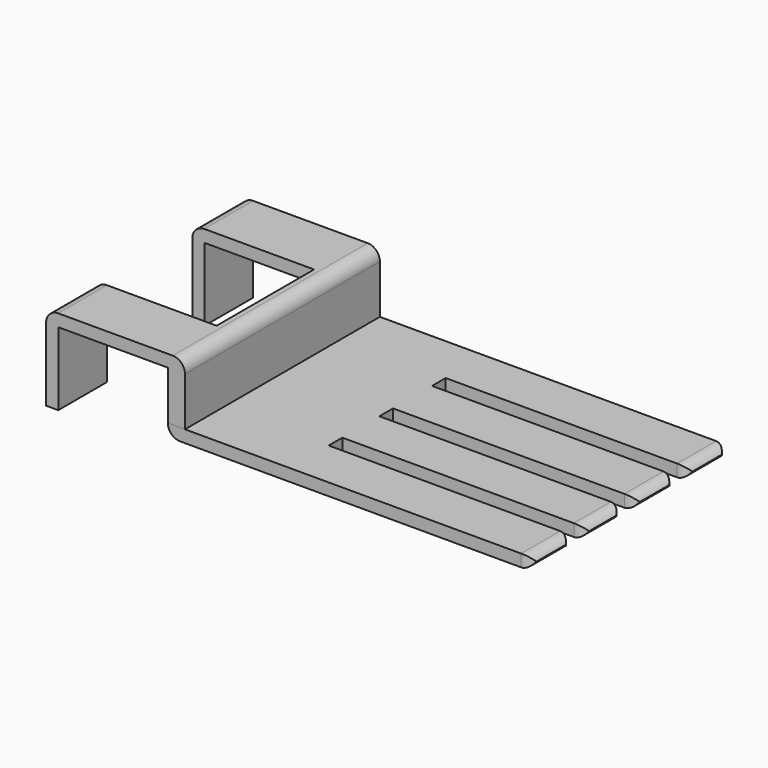
from build123d import *

# Parameters (mm, degrees)
F0_W         = 150
F0_H         = 100
F1_DEPTH     = 5
F2_W         = 100
F2_H         = 7
F3_DEPTH     = 5.001
F4_W         = 7
F4_H         = 100
F5_DEPTH     = 25
F6_W         = 25
F6_H         = 5
F7_DEPTH     = 50
F9_W         = 5
F9_H         = 25
F8_W         = 5
F8_H         = 25
F10_DEPTH    = 30
F11_R        = 4.99999
F11_2_R      = 4.99999
F12_T1_DEPTH = 45
F12_T3_DEPTH = 30
F12_T5_DEPTH = 44
F12_T7_DEPTH = 45
F12_T9_DEPTH = 45


# Not quite as in the source:
# - a fillet or chamfer that OpenCascade refuses, or shapes differently, is made with other operations: its cross-section is extruded or revolved along the edge and cut away or added
# - a fillet or chamfer is up to 0.001 mm smaller than in the source, because OpenCascade refuses the exact size


with BuildPart() as f1:
    # F0 (on Top) → F1 (new body)
    with BuildSketch(Plane.XY):
        with Locations((-2.425318882, 2.1896716207)):
            Rectangle(F0_W, F0_H)
    extrude(amount=F1_DEPTH)

    # F2 (on face) → F3 (cut, through all)
    with BuildSketch(Plane.XY.offset(5)):
        with Locations((22.574681118, 28.6896716207)):
            Rectangle(F2_W, F2_H)
        with Locations((22.574681118, 1.6896716207)):
            Rectangle(F2_W, F2_H)
        with Locations((22.574681118, -24.3103283793)):
            Rectangle(F2_W, F2_H)
    extrude(amount=-F3_DEPTH, mode=Mode.SUBTRACT)

    # F11#2 (radius 5 in the source; OpenCascade refuses exactly that, so slightly less here)
    f11_2_edges = [f1.edges().sort_by_distance(p)[0] for p in [
        (-77.425319, 2.189672, 0),
    ]]
    fillet(f11_2_edges, radius=F11_2_R)

    # F12: fillet of radius 5 on 16 edges, made by hand

    # F12_s2 → F12_t1 (cut)
    with BuildSketch(Plane.XZ.offset(15.3103283793)):
        with BuildLine():
            ThreePointArc((67.574681118, 0), (71.110215024, 1.4644660941), (72.574681118, 5))
            Line((72.574681118, 5), (72.574681118, 0))
            Line((72.574681118, 0), (67.574681118, 0))
        make_face()
        with BuildLine():
            ThreePointArc((67.574681118, 5), (71.110215024, 3.5355339059), (72.574681118, 0))
            Line((72.574681118, 0), (72.574681118, 5))
            Line((72.574681118, 5), (67.574681118, 5))
        make_face()
    extrude(amount=F12_T1_DEPTH, mode=Mode.SUBTRACT)

    # F12_s4 → F12_t3 (cut)
    with BuildSketch(Plane.XY.offset(-12.5)):
        with BuildLine():
            ThreePointArc((67.574681118, -27.8103283793), (71.110215024, -29.2747944733), (72.574681118, -32.8103283793))
            Line((72.574681118, -32.8103283793), (72.574681118, -27.8103283793))
            Line((72.574681118, -27.8103283793), (67.574681118, -27.8103283793))
        make_face()
        with BuildLine():
            ThreePointArc((67.574681118, -47.8103283793), (71.110215024, -46.3458622852), (72.574681118, -42.8103283793))
            Line((72.574681118, -42.8103283793), (72.574681118, -47.8103283793))
            Line((72.574681118, -47.8103283793), (67.574681118, -47.8103283793))
        make_face()
        with BuildLine():
            ThreePointArc((67.574681118, -1.8103283793), (71.110215024, -3.2747944733), (72.574681118, -6.8103283793))
            Line((72.574681118, -6.8103283793), (72.574681118, -1.8103283793))
            Line((72.574681118, -1.8103283793), (67.574681118, -1.8103283793))
        make_face()
        with BuildLine():
            ThreePointArc((72.574681118, -15.8103283793), (71.110215024, -19.3458622852), (67.574681118, -20.8103283793))
            Line((67.574681118, -20.8103283793), (72.574681118, -20.8103283793))
            Line((72.574681118, -20.8103283793), (72.574681118, -15.8103283793))
        make_face()
        with BuildLine():
            ThreePointArc((67.574681118, 25.1896716207), (71.110215024, 23.7252055267), (72.574681118, 20.1896716207))
            Line((72.574681118, 20.1896716207), (72.574681118, 25.1896716207))
            Line((72.574681118, 25.1896716207), (67.574681118, 25.1896716207))
        make_face()
        with BuildLine():
            ThreePointArc((72.574681118, 10.1896716207), (71.110215024, 6.6541377148), (67.574681118, 5.1896716207))
            Line((67.574681118, 5.1896716207), (72.574681118, 5.1896716207))
            Line((72.574681118, 5.1896716207), (72.574681118, 10.1896716207))
        make_face()
        with BuildLine():
            ThreePointArc((67.574681118, 52.1896716207), (71.110215024, 50.7252055267), (72.574681118, 47.1896716207))
            Line((72.574681118, 47.1896716207), (72.574681118, 52.1896716207))
            Line((72.574681118, 52.1896716207), (67.574681118, 52.1896716207))
        make_face()
        with BuildLine():
            ThreePointArc((72.574681118, 37.1896716207), (71.110215024, 33.6541377148), (67.574681118, 32.1896716207))
            Line((67.574681118, 32.1896716207), (72.574681118, 32.1896716207))
            Line((72.574681118, 32.1896716207), (72.574681118, 37.1896716207))
        make_face()
    extrude(amount=F12_T3_DEPTH, mode=Mode.SUBTRACT)

    # F12_s6 → F12_t5 (cut)
    with BuildSketch(Plane.XZ.offset(-10.6896716207)):
        with BuildLine():
            ThreePointArc((67.574681118, 0), (71.110215024, 1.4644660941), (72.574681118, 5))
            Line((72.574681118, 5), (72.574681118, 0))
            Line((72.574681118, 0), (67.574681118, 0))
        make_face()
        with BuildLine():
            ThreePointArc((67.574681118, 5), (71.110215024, 3.5355339059), (72.574681118, 0))
            Line((72.574681118, 0), (72.574681118, 5))
            Line((72.574681118, 5), (67.574681118, 5))
        make_face()
    extrude(amount=F12_T5_DEPTH, mode=Mode.SUBTRACT)

    # F12_s8 → F12_t7 (cut)
    with BuildSketch(Plane.XZ.offset(-37.6896716207)):
        with BuildLine():
            ThreePointArc((67.574681118, 0), (71.110215024, 1.4644660941), (72.574681118, 5))
            Line((72.574681118, 5), (72.574681118, 0))
            Line((72.574681118, 0), (67.574681118, 0))
        make_face()
        with BuildLine():
            ThreePointArc((67.574681118, 5), (71.110215024, 3.5355339059), (72.574681118, 0))
            Line((72.574681118, 0), (72.574681118, 5))
            Line((72.574681118, 5), (67.574681118, 5))
        make_face()
    extrude(amount=F12_T7_DEPTH, mode=Mode.SUBTRACT)

    # F12_s10 → F12_t9 (cut)
    with BuildSketch(Plane.XZ.offset(-64.6896716207)):
        with BuildLine():
            ThreePointArc((67.574681118, 0), (71.110215024, 1.4644660941), (72.574681118, 5))
            Line((72.574681118, 5), (72.574681118, 0))
            Line((72.574681118, 0), (67.574681118, 0))
        make_face()
        with BuildLine():
            ThreePointArc((67.574681118, 5), (71.110215024, 3.5355339059), (72.574681118, 0))
            Line((72.574681118, 0), (72.574681118, 5))
            Line((72.574681118, 5), (67.574681118, 5))
        make_face()
    extrude(amount=F12_T9_DEPTH, mode=Mode.SUBTRACT)


with BuildPart() as f5:
    # F4 (on face) → F5 (new body)
    with BuildSketch(Plane.XY.offset(5)):
        with Locations((-73.925318882, 2.1896716207)):
            Rectangle(F4_W, F4_H)
    extrude(amount=F5_DEPTH)

    # F6 (on face) → F7 (join)
    with BuildSketch(Plane(origin=(-77.425318882, 0, 0), x_dir=(0, -1, 0), z_dir=(-1, 0, 0))):
        with Locations((-39.6896716207, 27.5)):
            Rectangle(F6_W, F6_H)
        with Locations((35.3103283793, 27.5)):
            Rectangle(F6_W, F6_H)
    extrude(amount=F7_DEPTH)

    # F9 (on face) + F8 (on face) → F10 (join)
    with BuildSketch(Plane(origin=(0, 0, 25), x_dir=(1, 0, 0), z_dir=(0, 0, -1))):
        with Locations((-124.925318882, 35.3103283793)):
            Rectangle(F9_W, F9_H)
    with BuildSketch(Plane(origin=(0, 0, 25), x_dir=(1, 0, 0), z_dir=(0, 0, -1))):
        with Locations((-124.925318882, -39.6896716207)):
            Rectangle(F8_W, F8_H)
    extrude(amount=F10_DEPTH)

    # F11 (radius 5 in the source; OpenCascade refuses exactly that, so slightly less here)
    f11_edges = [f5.edges().sort_by_distance(p)[0] for p in [
        (-127.425319, 39.689672, 30),
        (-127.425319, -35.310328, 30),
        (-70.425319, 2.189672, 30),
    ]]
    fillet(f11_edges, radius=F11_R)


solid = Compound([f1.part, f5.part])
